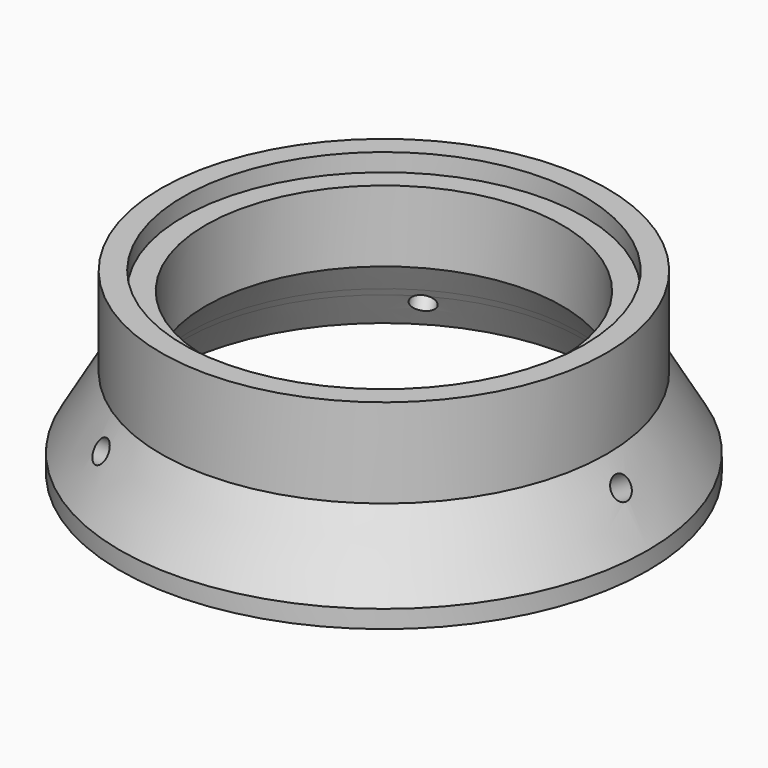
from build123d import *

# Parameters (mm, degrees)
F4_D            = 2.5781
F4_COPIES_COUNT = 3
F7_W            = 1.5
F7_H            = 2
F8_DEPTH        = 25


# Not quite as in the source:
# - a pattern or mirror of a feature is missing from the dataset's text; its kind, count and spacing are read off the source's solid


with BuildPart() as f1:
    # F0 (on Front) → F1 (revolve)
    with BuildSketch(Plane.XZ):
        Polygon((22.5, 18), (20, 18), (20, 10), (21.8094010768, 6.8660254038), (22.3094010768, 6), (24.6188021535, 2), (29.6188021535, 0), (29.6188021535, 2), (25, 10), (25, 18), (25, 20), (22.5, 20), align=None)
    revolve(axis=Axis((0, 0, 41.8434557322), (0, 0, 1)))

    # F4 (through all)
    with Locations(Plane(origin=(23.0801270189, 0, 13.3253175473), x_dir=(0, 1, 0), z_dir=(0.8660254038, 0, 0.5))):
        with Locations((0, -7.0773502692)):
            f4 = Hole(F4_D / 2)

    # F4_copies: F4 ×3 about axis
    f4_copies_axis = Axis((0, 0, 0), (0, 0, 1))
    for i in range(1, F4_COPIES_COUNT):
        add(f4.rotate(f4_copies_axis, i * 360 / F4_COPIES_COUNT), mode=Mode.SUBTRACT)

    # F7 (on line) → F8 (cut)
    with BuildSketch(Plane(origin=(0, 29.619, 0), x_dir=(-1, 0, 0), z_dir=(0, 1, 0))):
        Rectangle(F7_W, F7_H)
        with BuildLine():
            Line((-0.75, 1), (0.75, 1))
            ThreePointArc((0.75, 1), (0, 1.75), (-0.75, 1))
        make_face()
    extrude(amount=-F8_DEPTH, mode=Mode.SUBTRACT)


solid = f1.part
